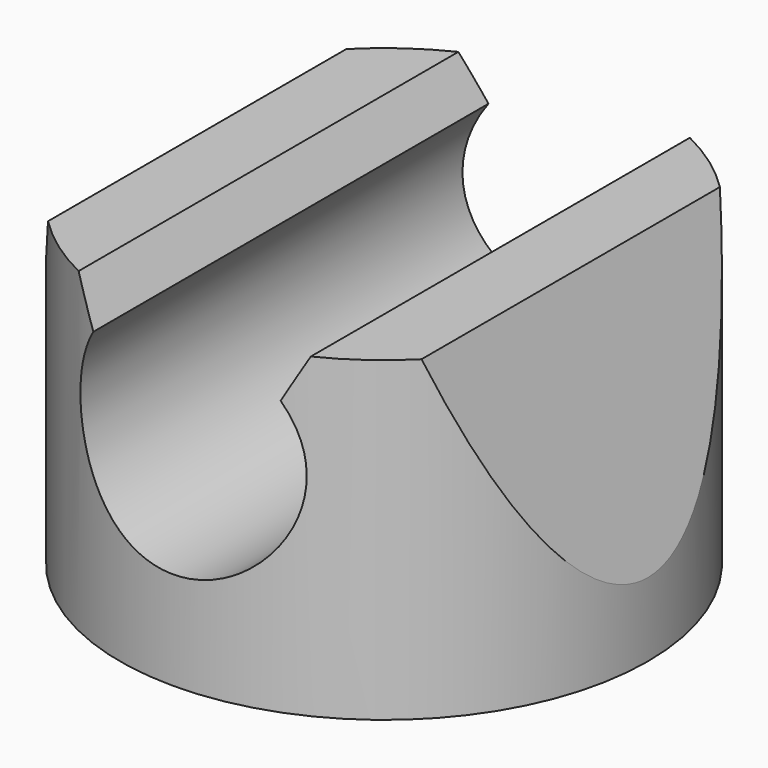
from build123d import *

# Parameters (mm, degrees)
F0_R        = 12.5
F1_DEPTH    = 15
F2_R        = 5.35
F3_DEPTH    = 19.7
F4_R        = 11.5
F5_DEPTH    = 2
F6_T1_DEPTH = 43.3845163924
F6_T3_DEPTH = 43.3709168199
F8_DEPTH    = 41


# Not quite as in the source:
# - a fillet or chamfer that OpenCascade refuses, or shapes differently, is made with other operations: its cross-section is extruded or revolved along the edge and cut away or added


with BuildPart() as f1:
    # F0 (on Top) → F1 (new body)
    with BuildSketch(Plane.XY):
        Circle(F0_R)
    extrude(amount=F1_DEPTH)

    # F2 (on Front) → F3 (cut, symmetric)
    with BuildSketch(Plane.XZ):
        with Locations((0.0221527088, 9.997321542)):
            Circle(F2_R)
    extrude(amount=F3_DEPTH, both=True, mode=Mode.SUBTRACT)

    # F4 (on Top) → F5 (cut)
    with BuildSketch(Plane.XY):
        Circle(F4_R)
    extrude(amount=F5_DEPTH, mode=Mode.SUBTRACT)

    # F6: chamfer of 7 on 2 edges, made by hand

    # F6_s2 → F6_t1 (cut)
    with BuildSketch(Plane.XZ.offset(-21.6922581962)):
        with BuildLine():
            Line((-4.2755328164, 12.7512221633), (-5.5992962087, 15.2473673359))
            Line((-5.5992962087, 15.2473673359), (-5.5992962087, 15.3873673359))
            ThreePointArc((-5.5992962087, 15.3873673359), (-3.7366893911, 15.14), (-1.8740825735, 15.14))
            Line((-1.8740825735, 15.14), (-1.8244614633, 14.869088788))
            ThreePointArc((-1.8244614633, 14.869088788), (-3.2288770936, 14.0685504994), (-4.1596371494, 12.6726843102))
            Line((-4.1596371494, 12.6726843102), (-4.2755328164, 12.7512221633))
        make_face()
    extrude(amount=F6_T1_DEPTH, mode=Mode.SUBTRACT)

    # F6_s4 → F6_t3 (cut)
    with BuildSketch(Plane.XZ.offset(-21.6854584099)):
        with BuildLine():
            Line((5.6436016264, 15.2473673359), (4.3198382341, 12.7512221633))
            Line((4.3198382341, 12.7512221633), (4.2039425671, 12.6726843102))
            ThreePointArc((4.2039425671, 12.6726843102), (3.2731825113, 14.0685504994), (1.868766881, 14.869088788))
            Line((1.868766881, 14.869088788), (1.9183879912, 15.14))
            ThreePointArc((1.9183879912, 15.14), (3.7809948088, 15.14), (5.6436016264, 15.3873673359))
            Line((5.6436016264, 15.3873673359), (5.6436016264, 15.2473673359))
        make_face()
    extrude(amount=F6_T3_DEPTH, mode=Mode.SUBTRACT)

    # F7 (on Front) → F8 (cut, symmetric)
    with BuildSketch(Plane.XZ):
        Polygon((22.090458405, 20.6357296556), (7.1151317097, 20.4473696649), (14.5756583661, -3.0394739006), align=None)
        Polygon((-14.5756583661, -3.0394739006), (-7.1151317097, 20.4473696649), (-22.090458405, 20.6357296556), align=None)
    extrude(amount=F8_DEPTH, both=True, mode=Mode.SUBTRACT)


solid = f1.part
